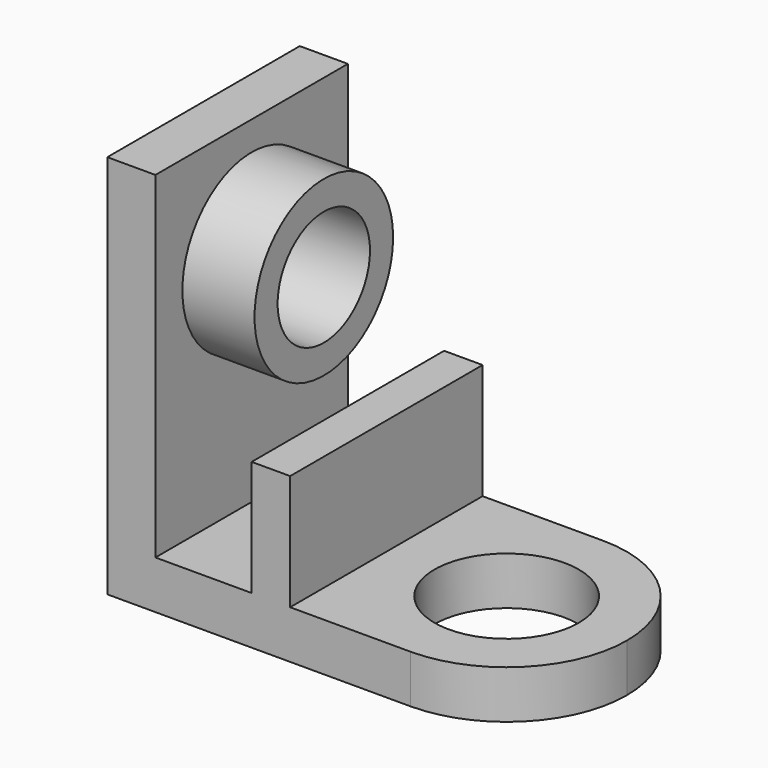
from build123d import *

# Parameters (mm, degrees)
F1_DEPTH = 50
F2_R     = 24.99999
F3_R     = 15
F4_DEPTH = 10
F5_R     = 18
F6_DEPTH = 15
F7_R     = 12
F8_DEPTH = 25


# Not quite as in the source:
# - a fillet or chamfer is up to 0.001 mm smaller than in the source, because OpenCascade refuses the exact size


with BuildPart() as f1:
    # F0 (on Front) → F1 (new body)
    with BuildSketch(Plane.XZ):
        Polygon((0, 80), (0, 0), (88, 0), (88, 10), (38, 10), (38, 34), (30, 34), (30, 10), (10, 10), (10, 80), align=None)
    extrude(amount=F1_DEPTH)

    # F2 (radius 25 in the source; OpenCascade refuses exactly that, so slightly less here)
    f2_edges = [f1.edges().sort_by_distance(p)[0] for p in [
        (88, -50, 5),
        (88, 0, 5),
    ]]
    fillet(f2_edges, radius=F2_R)

    # F3 (on face) → F4 (cut, through all)
    with BuildSketch(Plane.XY.offset(10)):
        with Locations((63, -25)):
            Circle(F3_R)
    extrude(amount=-F4_DEPTH, mode=Mode.SUBTRACT)

    # F5 (on face) → F6 (join)
    with BuildSketch(Plane.YZ.offset(10)):
        with Locations((-25, 56)):
            Circle(F5_R)
    extrude(amount=F6_DEPTH)

    # F7 (on face) → F8 (cut, through all)
    with BuildSketch(Plane.YZ.offset(25)):
        with Locations((-25, 56)):
            Circle(F7_R)
    extrude(amount=-F8_DEPTH, mode=Mode.SUBTRACT)


solid = f1.part
